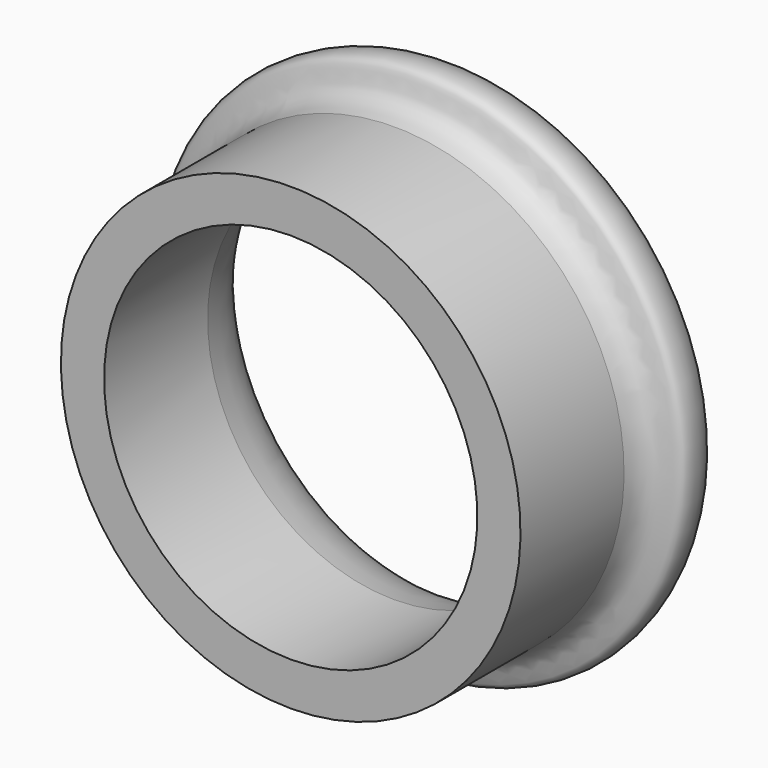
from build123d import *


with BuildPart() as f2:
    # F0 (on Right) → F2 (revolve)
    with BuildSketch(Plane.YZ):
        with BuildLine():
            Line((-12.3609009758, -43.25), (-12.3609009758, -53.25))
            Line((-12.3609009758, -53.25), (17.6390990242, -53.25))
            add(Edge.make_bspline(
                [(17.618613781, -43.25), (31.8222021326, -44.8877685905), (42.0131757878, -59.1744012288), (21.0233819627, -64.2057192342), (25.0903449501, -54.5590444197), (17.6390990242, -53.25)],
                knots=[0, 0, 0, 0, 0.4236601599, 0.7086548564, 1, 1, 1, 1], degree=3))
            Line((17.618613781, -43.25), (-12.3609009758, -43.25))
        make_face()
    revolve(axis=Axis((0, 37.7449579537, 0), (0, 1, 0)))


solid = f2.part
